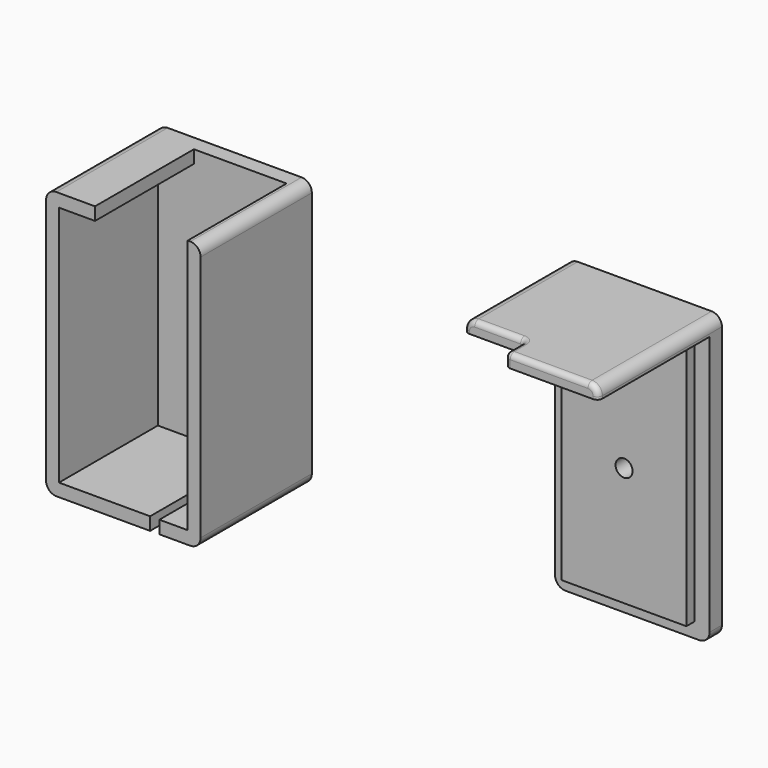
from build123d import *

# Parameters (mm, degrees)
F0_W      = 25
F0_H      = 47
F1_DEPTH  = 27
F0_R      = 1.65
F2_DEPTH  = 3
F3_W      = 1.8
F3_H      = 20
F4_DEPTH  = 25
F5_W      = 18
F5_H      = 24
F6_DEPTH  = 25
F8_DEPTH  = 3
F7_R      = 1.65
F9_DEPTH  = 5
F10_DEPTH = 30
F7_W      = 9
F7_H      = 2.5
F11_DEPTH = 25
F12_R     = 1


with BuildPart() as f1:
    # F0 (on Front) → F1 (new body)
    with BuildSketch(Plane.XZ):
        with BuildLine():
            Line((-28, 0), (-2, 0))
            ThreePointArc((-2, 0), (-0.5857864376, 0.5857864376), (0, 2))
            Line((0, 2), (0, 50))
            ThreePointArc((0, 50), (-0.5857864376, 51.4142135624), (-2, 52))
            Line((-2, 52), (-28, 52))
            ThreePointArc((-28, 52), (-29.4142135624, 51.4142135624), (-30, 50))
            Line((-30, 50), (-30, 2))
            ThreePointArc((-30, 2), (-29.4142135624, 0.5857864376), (-28, 0))
        make_face()
        with Locations((-15, 26)):
            Rectangle(F0_W, F0_H, mode=Mode.SUBTRACT)
    extrude(amount=F1_DEPTH)

    # F0 (on Front) → F2 (join)
    with BuildSketch(Plane.XZ):
        with Locations((-15, 26)):
            Rectangle(F0_W, F0_H)
        with Locations((-15, 26)):
            Circle(F0_R, mode=Mode.SUBTRACT)
    extrude(amount=F2_DEPTH)

    # F3 (on face) → F4 (cut)
    with BuildSketch(Plane(origin=(0, 0, 0), x_dir=(1, 0, 0), z_dir=(0, 0, -1))):
        with Locations((-8.9, 17)):
            Rectangle(F3_W, F3_H)
    extrude(amount=-F4_DEPTH, mode=Mode.SUBTRACT)

    # F5 (on face) → F6 (cut)
    with BuildSketch(Plane.XY.offset(52)):
        with Locations((-11.5, -15)):
            Rectangle(F5_W, F5_H)
    extrude(amount=-F6_DEPTH, mode=Mode.SUBTRACT)


with BuildPart() as f8:
    # F7 (on Front) → F8 (new body)
    with BuildSketch(Plane.XZ):
        with BuildLine():
            ThreePointArc((49.6213248736, 2), (50.2071113112, 0.5857864376), (51.6213248736, 0))
            Line((51.6213248736, 0), (77.6213248736, 0))
            ThreePointArc((77.6213248736, 0), (79.035538436, 0.5857864376), (79.6213248736, 2))
            Line((79.6213248736, 2), (79.6213248736, 50))
            Line((79.6213248736, 50), (79.6213248736, 52))
            Line((79.6213248736, 52), (79.6213248736, 52.5))
            Line((79.6213248736, 52.5), (76.7213248736, 52.5))
            Line((76.7213248736, 52.5), (76.7213248736, 49.1))
            Line((76.7213248736, 49.1), (76.7213248736, 2.9))
            Line((76.7213248736, 2.9), (52.5213248736, 2.9))
            Line((52.5213248736, 2.9), (52.5213248736, 49.1))
            Line((52.5213248736, 49.1), (52.5213248736, 52))
            Line((52.5213248736, 52), (52.5213248736, 52.5))
            Line((52.5213248736, 52.5), (49.6213248736, 52.5))
            Line((49.6213248736, 52.5), (49.6213248736, 52))
            Line((49.6213248736, 52), (49.6213248736, 50))
            Line((49.6213248736, 50), (49.6213248736, 2))
        make_face()
    extrude(amount=F8_DEPTH)

    # F7 (on Front) → F9 (join)
    with BuildSketch(Plane.XZ):
        Polygon((61.5213248736, 52.5), (52.5213248736, 52.5), (52.5213248736, 52), (52.5213248736, 49.1), (52.5213248736, 2.9), (76.7213248736, 2.9), (76.7213248736, 49.1), (76.7213248736, 52.5), align=None)
        with Locations((64.6213248736, 26)):
            Circle(F7_R, mode=Mode.SUBTRACT)
    extrude(amount=F9_DEPTH)

    # F7 (on Front) → F10 (join)
    with BuildSketch(Plane.XZ):
        with BuildLine():
            Line((76.7213248736, 52.5), (79.6213248736, 52.5))
            Line((79.6213248736, 52.5), (79.6213248736, 53))
            ThreePointArc((79.6213248736, 53), (79.035538436, 54.4142135624), (77.6213248736, 55))
            Line((77.6213248736, 55), (61.5213248736, 55))
            Line((61.5213248736, 55), (61.5213248736, 52.5))
            Line((61.5213248736, 52.5), (76.7213248736, 52.5))
        make_face()
    extrude(amount=F10_DEPTH)

    # F7 (on Front) → F11 (join)
    with BuildSketch(Plane.XZ):
        with Locations((57.0213248736, 53.75)):
            Rectangle(F7_W, F7_H)
        with BuildLine():
            Line((49.6213248736, 53), (49.6213248736, 52.5))
            Line((49.6213248736, 52.5), (52.5213248736, 52.5))
            Line((52.5213248736, 52.5), (52.5213248736, 55))
            Line((52.5213248736, 55), (51.6213248736, 55))
            ThreePointArc((51.6213248736, 55), (50.2071113112, 54.4142135624), (49.6213248736, 53))
        make_face()
    extrude(amount=F11_DEPTH)

    # F12
    f12_edges = [f8.edges().sort_by_distance(p)[0] for p in [
        (61.521325, -25, 53.75),
        (61.521325, -30, 53.75),
        (50.207111, -25, 54.414214),
        (79.035538, -30, 54.414214),
        (49.621325, -25, 52.75),
        (79.621325, -30, 52.75),
        (69.571325, -30, 55),
        (61.521325, -27.5, 55),
        (56.571325, -25, 55),
    ]]
    fillet(f12_edges, radius=F12_R)


solid = Compound([f1.part, f8.part])
